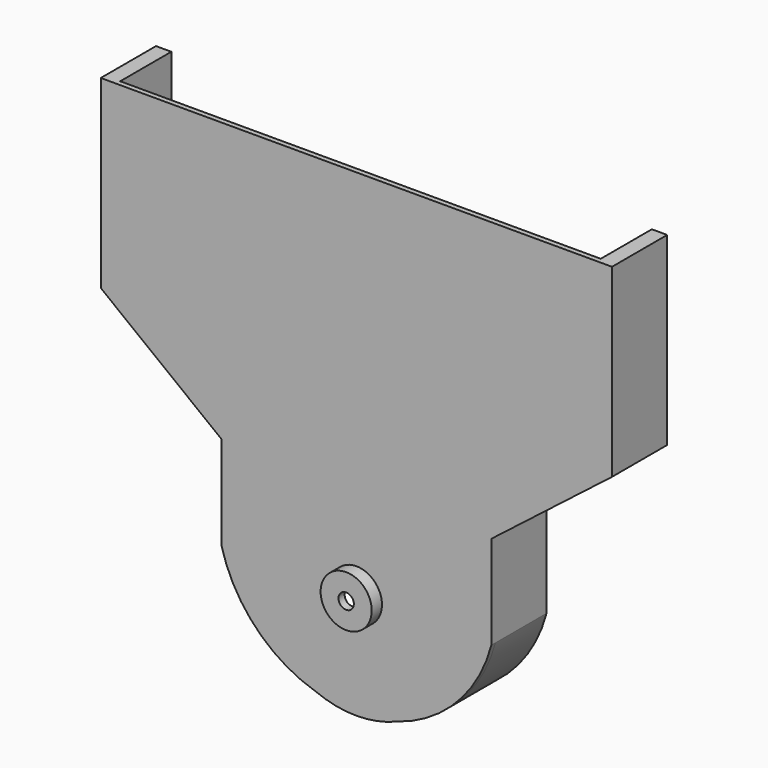
from build123d import *

# Parameters (mm, degrees)
F1_DEPTH  = 2
F2_R      = 10
F3_DEPTH  = 5
F4_R      = 8
F5_DEPTH  = 4
F6_R      = 3
F7_DEPTH  = 25
F9_DEPTH  = 25
F11_DEPTH = 25
F12_DEPTH = 25


# Not quite as in the source:
# - a feature names something its author has since deleted; it is built from what else it names


with BuildPart() as f1:
    # F0 (on Front) → F1 (new body)
    with BuildSketch(Plane.XZ):
        with BuildLine():
            Line((0, 0), (15.8813624432, -38.3410005992))
            ThreePointArc((15.8813624432, -38.3410005992), (41.5, 0), (15.8813624432, 38.3410005992))
            Line((15.8813624432, 38.3410005992), (0, 0))
        make_face()
        with BuildLine():
            ThreePointArc((0, -41.5), (8.0962483637, -40.7025891367), (15.8813624432, -38.3410005992))
            Line((15.8813624432, -38.3410005992), (0, 0))
            Line((0, 0), (0, -41.5))
        make_face()
        with BuildLine():
            ThreePointArc((15.8813624432, 38.3410005992), (41.5, 0), (15.8813624432, -38.3410005992))
            ThreePointArc((15.8813624432, -38.3410005992), (39.330613444, -23.9742260076), (52.803106606, 0))
            Line((52.803106606, 0), (52.803106606, 36.6300418973))
            Line((52.803106606, 36.6300418973), (100, 73.2887908816))
            Line((100, 73.2887908816), (100, 145.6475704908))
            Line((100, 145.6475704908), (0, 145.6475704908))
            Line((0, 145.6475704908), (-100, 145.6475704908))
            Line((-100, 145.6475704908), (-100, 73.2887908816))
            Line((-100, 73.2887908816), (-52.803106606, 36.6300418973))
            Line((-52.803106606, 36.6300418973), (-52.803106606, 0))
            ThreePointArc((-52.803106606, 0), (-39.330613444, -23.9742260076), (-15.8813624432, -38.3410005992))
            ThreePointArc((-15.8813624432, -38.3410005992), (-41.5, 0), (-15.8813624432, 38.3410005992))
            ThreePointArc((-15.8813624432, 38.3410005992), (0, 41.5), (15.8813624432, 38.3410005992))
        make_face()
        with BuildLine():
            Line((0, -41.5), (0, 0))
            Line((0, 0), (-15.8813624432, -38.3410005992))
            ThreePointArc((-15.8813624432, -38.3410005992), (-8.0962483637, -40.7025891367), (0, -41.5))
        make_face()
        with BuildLine():
            Line((-15.8813624432, -38.3410005992), (0, 0))
            Line((0, 0), (-15.8813624432, 38.3410005992))
            ThreePointArc((-15.8813624432, 38.3410005992), (-41.5, 0), (-15.8813624432, -38.3410005992))
        make_face()
        with BuildLine():
            Line((0, 0), (15.8813624432, 38.3410005992))
            ThreePointArc((15.8813624432, 38.3410005992), (0, 41.5), (-15.8813624432, 38.3410005992))
            Line((-15.8813624432, 38.3410005992), (0, 0))
        make_face()
    extrude(amount=F1_DEPTH)

    # F2 (on face) → F3 (join)
    with BuildSketch(Plane.XZ.offset(2)):
        Circle(F2_R)
    extrude(amount=F3_DEPTH)

    # F4 (on face) → F5 (cut)
    with BuildSketch(Plane(origin=(0, 0, 0), x_dir=(-1, 0, 0), z_dir=(0, 1, 0))):
        Circle(F4_R)
    extrude(amount=-F5_DEPTH, mode=Mode.SUBTRACT)

    # F6 (on face) → F7 (cut)
    with BuildSketch(Plane(origin=(0, 0, 0), x_dir=(-1, 0, 0), z_dir=(0, 1, 0))):
        Circle(F6_R)
    extrude(amount=-F7_DEPTH, mode=Mode.SUBTRACT)

    # F8 (on face) → F9 (join)
    with BuildSketch(Plane.XZ):
        with BuildLine():
            Line((100, 145.6475704908), (94, 145.6475704908))
            Line((94, 145.6475704908), (94, 73.2887908816))
            Line((94, 73.2887908816), (23.1737587601, 37.3859927058))
            ThreePointArc((23.1737587601, 37.3859927058), (38.7897108638, 21.4707349754), (44.803106606, 0))
            Line((44.803106606, 0), (52.803106606, 0))
            Line((52.803106606, 0), (52.803106606, 36.6300418973))
            Line((52.803106606, 36.6300418973), (100, 73.2887908816))
            Line((100, 73.2887908816), (100, 145.6475704908))
        make_face()
        with BuildLine():
            Line((-100, 145.6475704908), (-100, 73.2887908816))
            Line((-100, 73.2887908816), (-52.803106606, 36.6300418973))
            Line((-52.803106606, 36.6300418973), (-52.803106606, 0))
            Line((-52.803106606, 0), (-44.803106606, 0))
            ThreePointArc((-44.803106606, 0), (-38.7897108638, 21.4707349754), (-23.1737587601, 37.3859927058))
            Line((-23.1737587601, 37.3859927058), (-94, 73.2887908816))
            Line((-94, 73.2887908816), (-94, 143.9662277699))
            Line((-94, 143.9662277699), (-94, 145.6475704908))
            Line((-94, 145.6475704908), (-100, 145.6475704908))
        make_face()
    extrude(amount=-F9_DEPTH)

    # F10 (on face) → F11 (join)
    with BuildSketch(Plane.XZ):
        with BuildLine():
            ThreePointArc((44.803106606, 0), (38.1524173859, -20.6793456236), (22.573144677, -35.8171547249))
            ThreePointArc((22.573144677, -35.8171547249), (41.7266336711, -21.3171100871), (52.803106606, 0))
            Line((52.803106606, 0), (44.803106606, 0))
        make_face()
    extrude(amount=-F11_DEPTH)

    # F10 (on face) → F12 (join)
    with BuildSketch(Plane.XZ):
        with BuildLine():
            ThreePointArc((-52.803106606, 0), (-41.7266336711, -21.3171100871), (-22.573144677, -35.8171547249))
            ThreePointArc((-22.573144677, -35.8171547249), (-38.1524173859, -20.6793456236), (-44.803106606, 0))
            Line((-44.803106606, 0), (-52.803106606, 0))
        make_face()
    extrude(amount=-F12_DEPTH)


solid = f1.part
